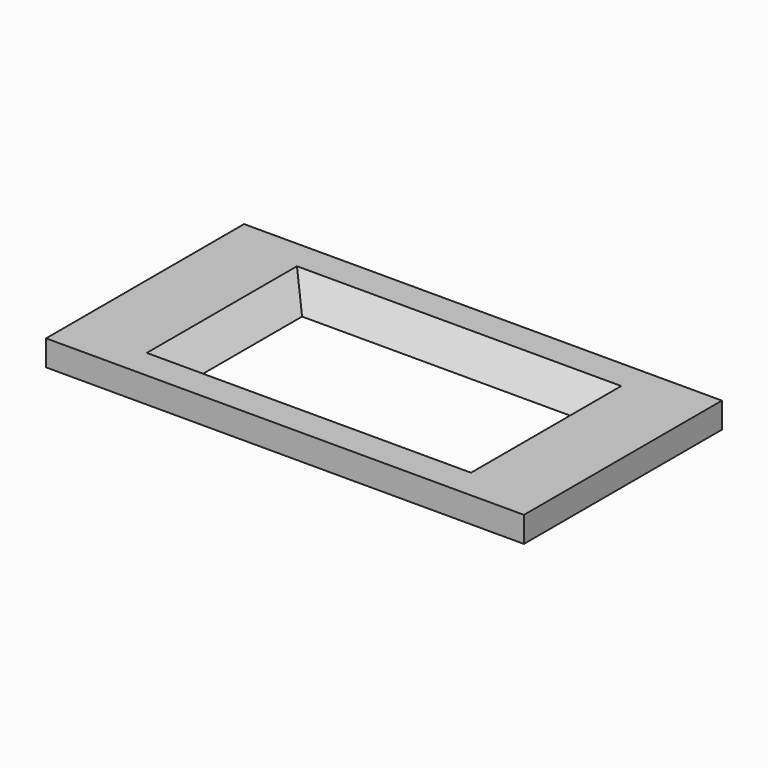
from build123d import *

# Parameters (mm, degrees)
F0_W     = 355.6
F0_H     = 184.15
F0_W_2   = 203.2
F0_H_2   = 101.6
F1_DEPTH = 19.05
F2_SIZE2 = 19.04999
F2_SIZE  = 19.04999


# Not quite as in the source:
# - a fillet or chamfer is up to 0.001 mm smaller than in the source, because OpenCascade refuses the exact size


with BuildPart() as f1:
    # F0 (on Top) → F1 (new body)
    with BuildSketch(Plane.XY):
        Rectangle(F0_W, F0_H)
        Rectangle(F0_W_2, F0_H_2, mode=Mode.SUBTRACT)
    extrude(amount=F1_DEPTH)

    # F2 (size 19.05 and 19.05 in the source; OpenCascade refuses exactly that, so slightly less here)
    f2_edges = [f1.edges().sort_by_distance(p)[0] for p in [
        (-101.6, 0, 19.05),
        (0, 50.8, 19.05),
        (101.6, 0, 19.05),
        (0, -50.8, 19.05),
    ]]
    chamfer(f2_edges, length=F2_SIZE, length2=F2_SIZE2)


solid = f1.part
